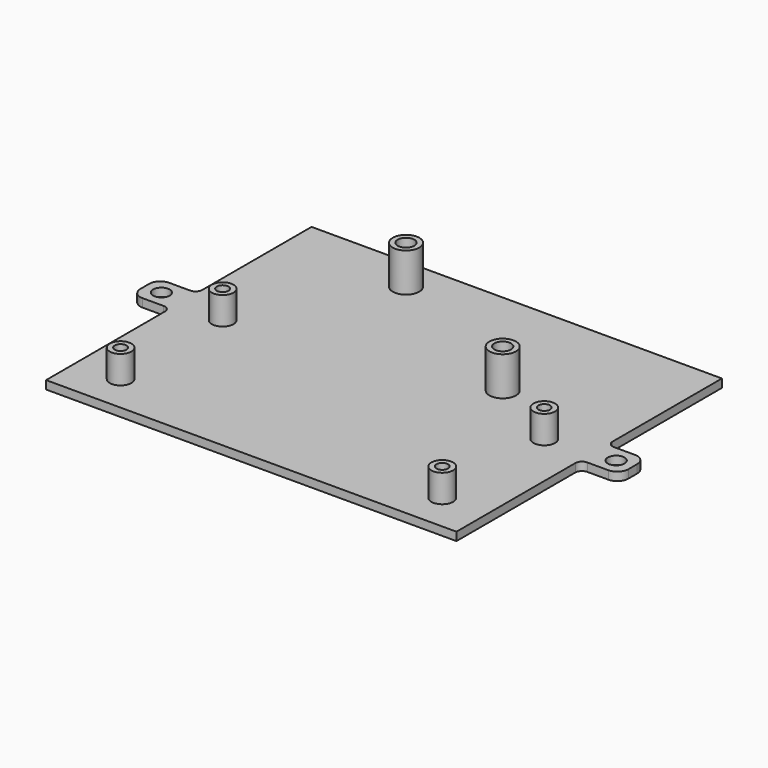
from build123d import *

# Parameters (mm, degrees)
F0_R     = 1.05
F0_R_2   = 1.5
F1_DEPTH = 1.5
F3_R     = 1.2
F4_R     = 1.95
F4_R_2   = 1.05
F5_DEPTH = 5
F4_R_3   = 2.4
F4_R_4   = 1.5
F6_DEPTH = 7


with BuildPart() as f1:
    # F0 (on Top) → F1 (new body)
    with BuildSketch(Plane.XY):
        Polygon((37, 30.5212866254), (-37, 30.5212866254), (-37, 4.6800224319), (-37, -1.3199775681), (-37, -29.3157063685), (37, -29.3157063685), (37, -1.3199775681), (37, 4.6800224319), align=None)
        with Locations((-29, -22.5189467669)):
            Circle(F0_R, mode=Mode.SUBTRACT)
        with Locations((-29, 0.4810532331)):
            Circle(F0_R, mode=Mode.SUBTRACT)
        with Locations((29, -22.5189467669)):
            Circle(F0_R, mode=Mode.SUBTRACT)
        with Locations((29, 0.4810532331)):
            Circle(F0_R, mode=Mode.SUBTRACT)
        with Locations((-15.2, 24.5643973112)):
            Circle(F0_R_2, mode=Mode.SUBTRACT)
        with Locations((15.2, 8.3643973112)):
            Circle(F0_R_2, mode=Mode.SUBTRACT)
        with BuildLine():
            Line((-37, -1.3199775681), (-37, 4.6800224319))
            Line((-37, 4.6800224319), (-42, 4.6800224319))
            ThreePointArc((-42, 4.6800224319), (-43.4142135624, 4.0942359942), (-44, 2.6800224319))
            Line((-44, 2.6800224319), (-44, 0.6800224319))
            ThreePointArc((-44, 0.6800224319), (-43.4142135624, -0.7341911305), (-42, -1.3199775681))
            Line((-42, -1.3199775681), (-37, -1.3199775681))
        make_face()
        with Locations((-41, 1.6800224319)):
            Circle(F0_R_2, mode=Mode.SUBTRACT)
        with BuildLine():
            Line((42, 4.6800224319), (37, 4.6800224319))
            Line((37, 4.6800224319), (37, -1.3199775681))
            Line((37, -1.3199775681), (42, -1.3199775681))
            ThreePointArc((42, -1.3199775681), (43.4142135624, -0.7341911305), (44, 0.6800224319))
            Line((44, 0.6800224319), (44, 2.6800224319))
            ThreePointArc((44, 2.6800224319), (43.4142135624, 4.0942359942), (42, 4.6800224319))
        make_face()
        with Locations((41, 1.6800224319)):
            Circle(F0_R_2, mode=Mode.SUBTRACT)
    extrude(amount=-F1_DEPTH)

    # F3
    f3_edges = [f1.edges().sort_by_distance(p)[0] for p in [
        (-37, -1.319978, -0.75),
        (-37, 4.680022, -0.75),
        (37, -1.319978, -0.75),
        (37, 4.680022, -0.75),
    ]]
    fillet(f3_edges, radius=F3_R)

    # F4 (on face) → F5 (join)
    with BuildSketch(Plane.XY):
        with Locations((-29, 0.4810532331)):
            Circle(F4_R)
        with Locations((-29, 0.4810532331)):
            Circle(F4_R_2, mode=Mode.SUBTRACT)
        with Locations((-29, -22.5189467669)):
            Circle(F4_R)
        with Locations((-29, -22.5189467669)):
            Circle(F4_R_2, mode=Mode.SUBTRACT)
        with Locations((29, -22.5189467669)):
            Circle(F4_R)
        with Locations((29, -22.5189467669)):
            Circle(F4_R_2, mode=Mode.SUBTRACT)
        with Locations((29, 0.4810532331)):
            Circle(F4_R)
        with Locations((29, 0.4810532331)):
            Circle(F4_R_2, mode=Mode.SUBTRACT)
    extrude(amount=F5_DEPTH)

    # F4 (on face) → F6 (join)
    with BuildSketch(Plane.XY):
        with Locations((-15.2, 24.5643973112)):
            Circle(F4_R_3)
        with Locations((-15.2, 24.5643973112)):
            Circle(F4_R_4, mode=Mode.SUBTRACT)
        with Locations((15.2, 8.3643973112)):
            Circle(F4_R_3)
        with Locations((15.2, 8.3643973112)):
            Circle(F4_R_4, mode=Mode.SUBTRACT)
    extrude(amount=F6_DEPTH)


solid = f1.part
